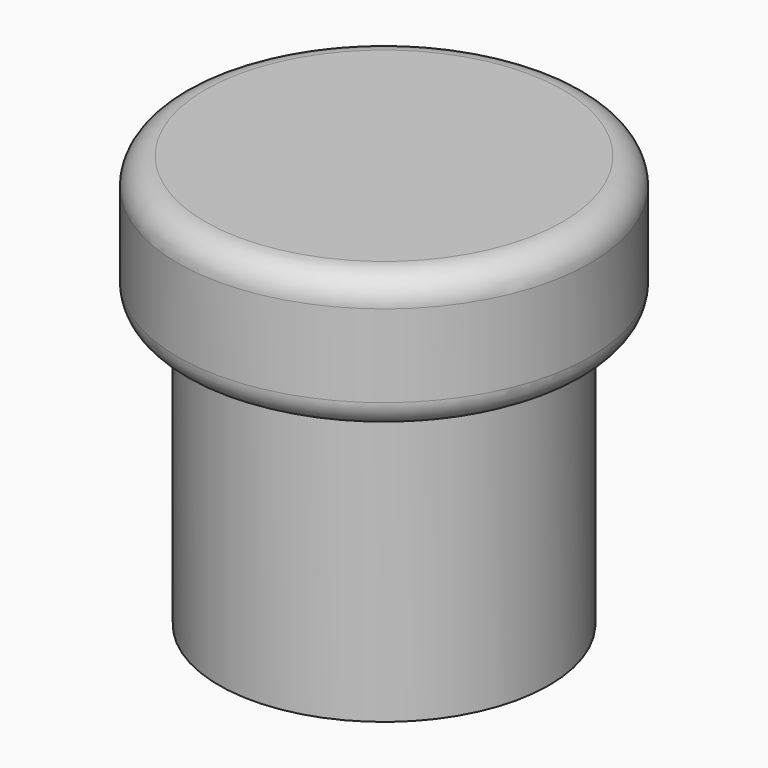
from build123d import *

# Parameters (mm, degrees)
F0_R     = 6
F1_DEPTH = 10
F2_R     = 7.5
F3_DEPTH = 5
F4_R     = 1


with BuildPart() as f1:
    # F0 (on Top) → F1 (new body)
    with BuildSketch(Plane.XY):
        Circle(F0_R)
    extrude(amount=F1_DEPTH)

    # F2 (on face) → F3 (join)
    with BuildSketch(Plane.XY.offset(10)):
        Circle(F2_R)
    extrude(amount=F3_DEPTH)

    # F4
    f4_edges = [f1.edges().sort_by_distance(p)[0] for p in [
        (-7.5, 0, 10),
        (-7.5, 0, 15),
    ]]
    fillet(f4_edges, radius=F4_R)


solid = f1.part
